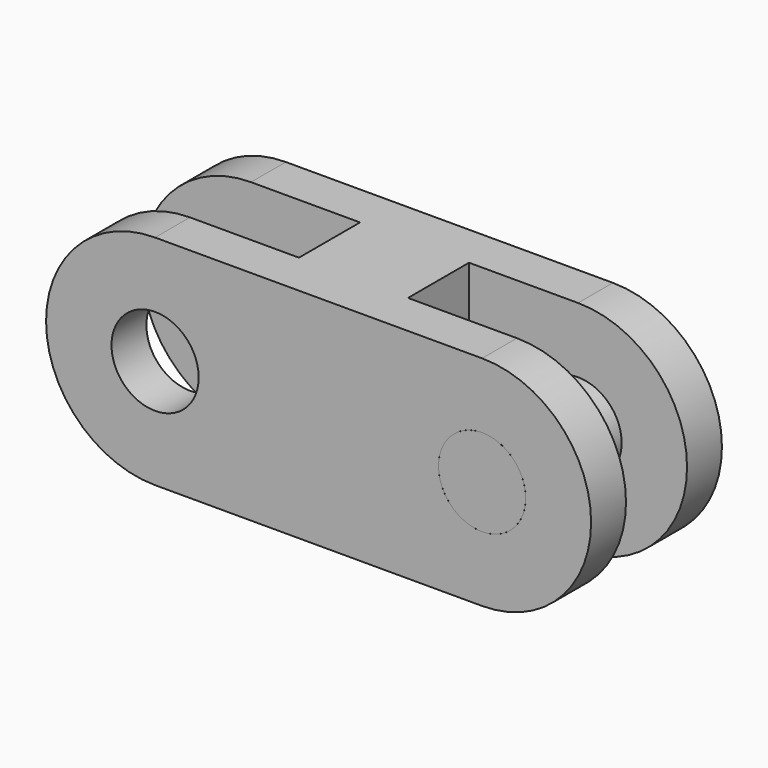
from build123d import *

# Parameters (mm, degrees)
F0_R     = 4
F1_DEPTH = 7.5
F2_W     = 13.542375192
F2_H     = 7
F2_W_2   = 10
F3_DEPTH = 20.001
F4_R     = 4
F5_DEPTH = 15


# Not quite as in the source:
# - a pattern or mirror of a feature is missing from the dataset's text; its kind, count and spacing are read off the source's solid


with BuildPart() as f1:
    # F0 (on Front) → F1 (new body, symmetric)
    with BuildSketch(Plane.XZ):
        with BuildLine():
            Line((15, 10), (-15, 10))
            ThreePointArc((-15, 10), (-25, 0), (-15, -10))
            Line((-15, -10), (15, -10))
            ThreePointArc((15, -10), (25, 0), (15, 10))
        make_face()
        with Locations((-15, 0)):
            Circle(F0_R, mode=Mode.SUBTRACT)
        with Locations((15, 0)):
            Circle(F0_R, mode=Mode.SUBTRACT)
    extrude(amount=F1_DEPTH, both=True)

    # F2 (on face) → F3 (cut, through all)
    with BuildSketch(Plane(origin=(0, 0, -10), x_dir=(1, 0, 0), z_dir=(0, 0, -1))):
        with Locations((21.771187596, 0)):
            Rectangle(F2_W, F2_H)
        with Locations((10, 0)):
            Rectangle(F2_W_2, F2_H)
    f3 = extrude(amount=-F3_DEPTH, mode=Mode.SUBTRACT)

    # F3_copies: F3 across plane
    add(f3.mirror(Plane(origin=(0, 0, 0), x_dir=(0, 0, -1), z_dir=(-1, 0, 0))), mode=Mode.SUBTRACT)


with BuildPart() as f5:
    # F4 (on face) → F5 (new body)
    with BuildSketch(Plane(origin=(0, 7.5, 0), x_dir=(-1, 0, 0), z_dir=(0, 1, 0))):
        with Locations((-15, 0)):
            Circle(F4_R)
    extrude(amount=-F5_DEPTH)


with BuildPart() as f5b:
    # F4 (on face) → F5, piece 2 (new body)
    with BuildSketch(Plane(origin=(0, 7.5, 0), x_dir=(-1, 0, 0), z_dir=(0, 1, 0))):
        with Locations((15, 0)):
            Circle(F4_R)
    extrude(amount=-F5_DEPTH)


solid = Compound([f1.part, f5.part])
